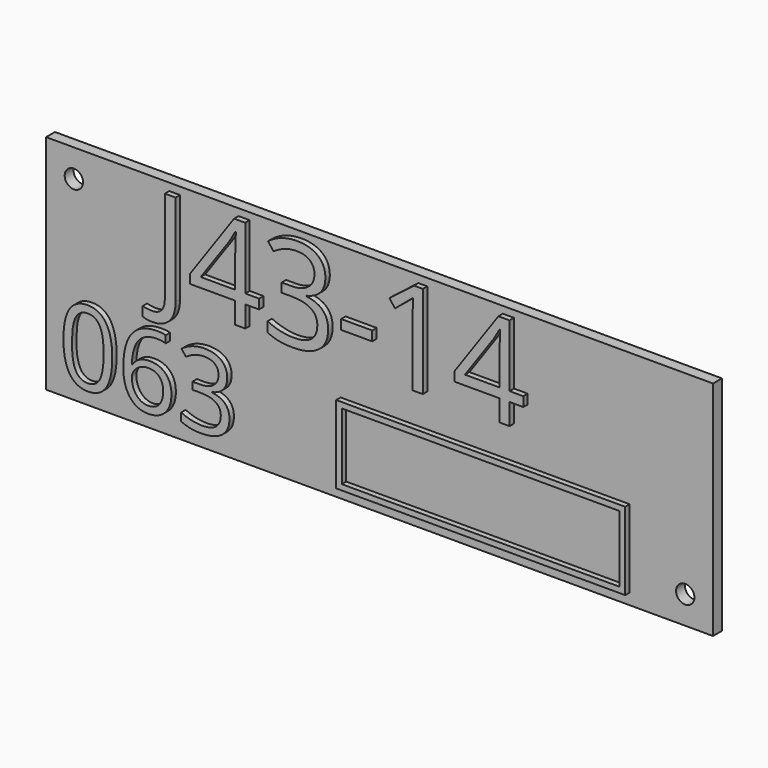
from build123d import *

# Parameters (mm, degrees)
F0_W         = 120
F0_H         = 40
F1_DEPTH     = 2
F3_D         = 3.3
F4_TEXT_SIZE = 23.3442759627
F5_DEPTH     = 1
F6_TEXT_SIZE = 18.5894526641
F7_DEPTH     = 1
F8_W         = 52
F8_H         = 14
F8_W_2       = 49.99999962
F8_H_2       = 11.99999962
F9_DEPTH     = 1


# Not quite as in the source:
# - Text() gives the source's letters only with a copy of the font that has no kerning and outlines rounded to 1/6400 em; it was checked with that copy


with BuildPart() as f1:
    # F0 (on Front) → F1 (new body)
    with BuildSketch(Plane.XZ):
        Rectangle(F0_W, F0_H)
    extrude(amount=F1_DEPTH)

    # F3 (through all)
    with Locations(Plane.XZ.offset(2)):
        with Locations((-55, 15), (55, -15)):
            Hole(F3_D / 2)

    # F4 (on face) → F5 (join)
    with BuildSketch(Plane.XZ.offset(2)):
        with Locations((-40, 2)):
            Text('J43-14', F4_TEXT_SIZE, font='Open Sans', text_align=(TextAlign.LEFT, TextAlign.BOTTOM))
    extrude(amount=F5_DEPTH)

    # F6 (on face) → F7 (join)
    with BuildSketch(Plane.XZ.offset(2)):
        with Locations((-57, -17)):
            Text('063', F6_TEXT_SIZE, font='Open Sans', text_align=(TextAlign.LEFT, TextAlign.BOTTOM))
    extrude(amount=F7_DEPTH)

    # F8 (on face) → F9 (join)
    with BuildSketch(Plane.XZ.offset(2)):
        with Locations((19, -11)):
            Rectangle(F8_W, F8_H)
        with Locations((19, -11)):
            Rectangle(F8_W_2, F8_H_2, mode=Mode.SUBTRACT)
    extrude(amount=F9_DEPTH)


solid = f1.part
